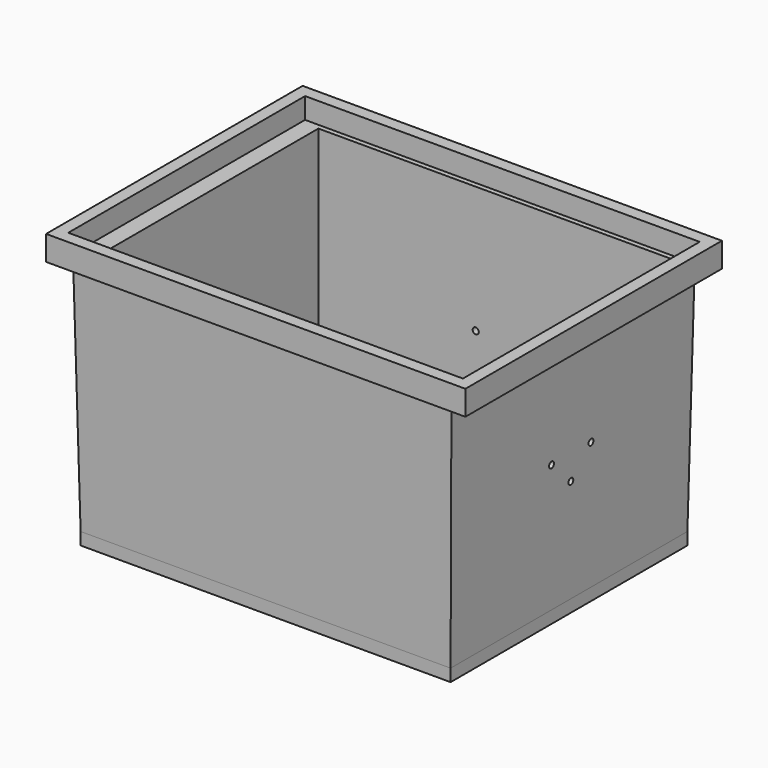
from build123d import *

# Parameters (mm, degrees)
F0_W                   = 381
F0_H                   = 304.8
F0_W_2                 = 370.84
F0_H_2                 = 294.64
F1_DEPTH               = 241.3
DRAFT_F1_DRAFTED_ANGLE = -1
F2_W                   = 431.8
F2_H                   = 330.2
F3_DEPTH               = 25.4
F4_W                   = 381
F4_H                   = 304.8
F5_DEPTH               = 12.7
F6_W                   = 406.4
F6_H                   = 304.8
F7_DEPTH               = 21.59
F8_W                   = 370.84
F8_H                   = 294.64
F9_DEPTH               = 245.111
F10_R                  = 3.175
F11_DEPTH              = 76.2
F13_R                  = 3.175
F14_DEPTH              = 528.321


# Not quite as in the source:
# - an extrude with a draft is written as a straight extrude whose walls are then drafted


with BuildPart() as f1:
    # F0 (on Top) → F1 (new body)
    with BuildSketch(Plane.XY):
        Rectangle(F0_W, F0_H)
        Rectangle(F0_W_2, F0_H_2, mode=Mode.SUBTRACT)
    extrude(amount=F1_DEPTH)

    # draft_F1_drafted
    draft_f1_drafted_walls = [f1.faces().sort_by_distance(p)[0] for p in [
        (0, 152.4, 160.8666666667),
        (-190.5, 0, 160.8666666667),
        (0, -152.4, 160.8666666667),
        (190.5, 0, 160.8666666667),
        (0, -147.32, 160.8666666667),
        (-185.42, 0, 160.8666666667),
        (0, 147.32, 160.8666666667),
        (185.42, 0, 160.8666666667),
    ]]
    draft(draft_f1_drafted_walls, neutral_plane=Plane.XY, angle=DRAFT_F1_DRAFTED_ANGLE)

    # F2 (on face) → F3 (join)
    with BuildSketch(Plane.XY.offset(241.3)):
        Rectangle(F2_W, F2_H)
    extrude(amount=F3_DEPTH)

    # F4 (on face) → F5 (join)
    with BuildSketch(Plane(origin=(0, 0, 0), x_dir=(1, 0, 0), z_dir=(0, 0, -1))):
        Rectangle(F4_W, F4_H)
    extrude(amount=F5_DEPTH)

    # F6 (on face) → F7 (cut)
    with BuildSketch(Plane.XY.offset(266.7)):
        Rectangle(F6_W, F6_H)
    extrude(amount=-F7_DEPTH, mode=Mode.SUBTRACT)

    # F8 (on face) → F9 (cut, through all)
    with BuildSketch(Plane.XY.offset(245.11)):
        Rectangle(F8_W, F8_H)
    extrude(amount=-F9_DEPTH, mode=Mode.SUBTRACT)

    # F10 (on face) → F11 (cut)
    with BuildSketch(Plane(origin=(0, 152.3535810189, -2.6593416487), x_dir=(-1, 0, 0), z_dir=(0, 0.9998476952, -0.0174524064))):
        with Locations((-116.2948438135, 116.9616810126)):
            Circle(F10_R)
        with Locations((-65.4948438135, 116.9616810126)):
            Circle(F10_R)
        with Locations((-27.3948438135, 116.9616810126)):
            Circle(F10_R)
        with Locations((23.4051561865, 116.9616810126)):
            Circle(F10_R)
        with Locations((-1.9948438135, 91.5616810126)):
            Circle(F10_R)
        with Locations((-90.8948438135, 91.5616810126)):
            Circle(F10_R)
    extrude(amount=-F11_DEPTH, mode=Mode.SUBTRACT)

    # F13 (on offset) → F14 (cut, through all)
    with BuildSketch(Plane(origin=(312.42, 0, 0), x_dir=(0, -1, 0), z_dir=(-1, 0, 0))):
        with Locations((-25.4, 133.35)):
            Circle(F13_R)
        with Locations((25.4, 133.35)):
            Circle(F13_R)
        with Locations((0, 107.95)):
            Circle(F13_R)
    extrude(amount=F14_DEPTH, mode=Mode.SUBTRACT)


solid = f1.part
